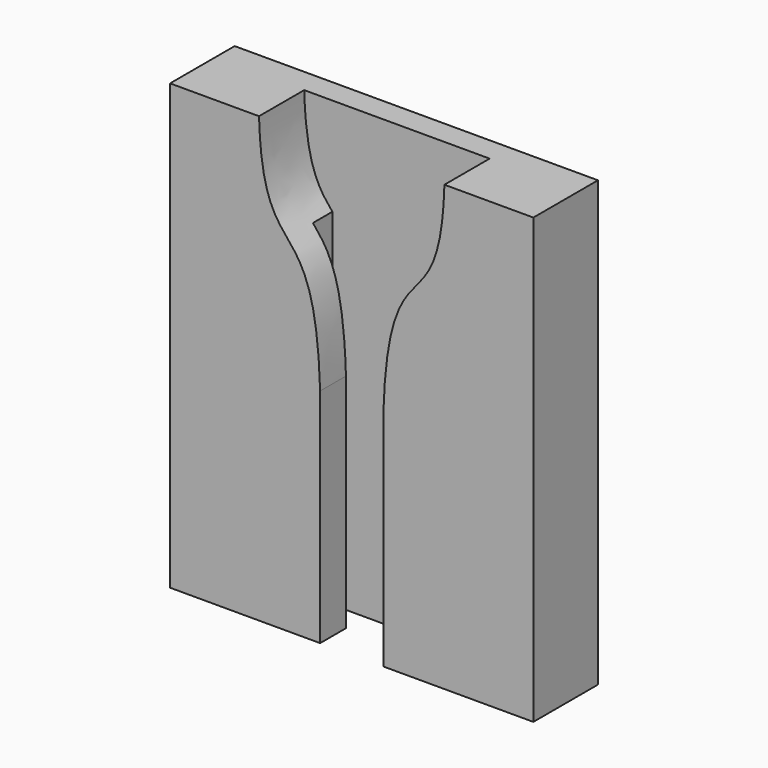
from build123d import *

# Parameters (mm, degrees)
F0_W     = 45
F0_H     = 55
F1_DEPTH = 10
F3_DEPTH = 7
F4_W     = 16
F4_H     = 3
F5_DEPTH = 55.0010001


with BuildPart() as f1:
    # F0 (on Front) → F1 (new body)
    with BuildSketch(Plane.XZ):
        Rectangle(F0_W, F0_H)
    extrude(amount=F1_DEPTH)

    # F2 (on face) → F3 (cut)
    with BuildSketch(Plane.XZ.offset(10)):
        with BuildLine():
            Line((3.9123152383, -27.5), (3.9123152383, 0))
            add(Edge.make_bspline(
                [(3.9123152383, 0), (4.5414378197, 20.6852698078), (10.9457386037, 10.2673236529), (11.484915749, 27.5)],
                knots=[0, 0, 0, 0, 28.5235740835, 28.5235740835, 28.5235740835, 28.5235740835], degree=3))
            Line((11.484915749, 27.5), (-11.484915749, 27.5))
            add(Edge.make_bspline(
                [(-3.9123152383, 0), (-4.5414378197, 20.6852698078), (-10.9457386037, 10.2673236529), (-11.484915749, 27.5)],
                knots=[0, 0, 0, 0, 28.5235740835, 28.5235740835, 28.5235740835, 28.5235740835], degree=3))
            Line((-3.9123152383, 0), (-3.9123152383, -27.5))
            Line((-3.9123152383, -27.5), (0, -27.5))
            Line((0, -27.5), (3.9123152383, -27.5))
        make_face()
    extrude(amount=-F3_DEPTH, mode=Mode.SUBTRACT)

    # F4 (on face) → F5 (cut, through all)
    with BuildSketch(Plane.XY.offset(27.5)):
        with Locations((0, -4.5)):
            Rectangle(F4_W, F4_H)
    extrude(amount=-F5_DEPTH, mode=Mode.SUBTRACT)


solid = f1.part
